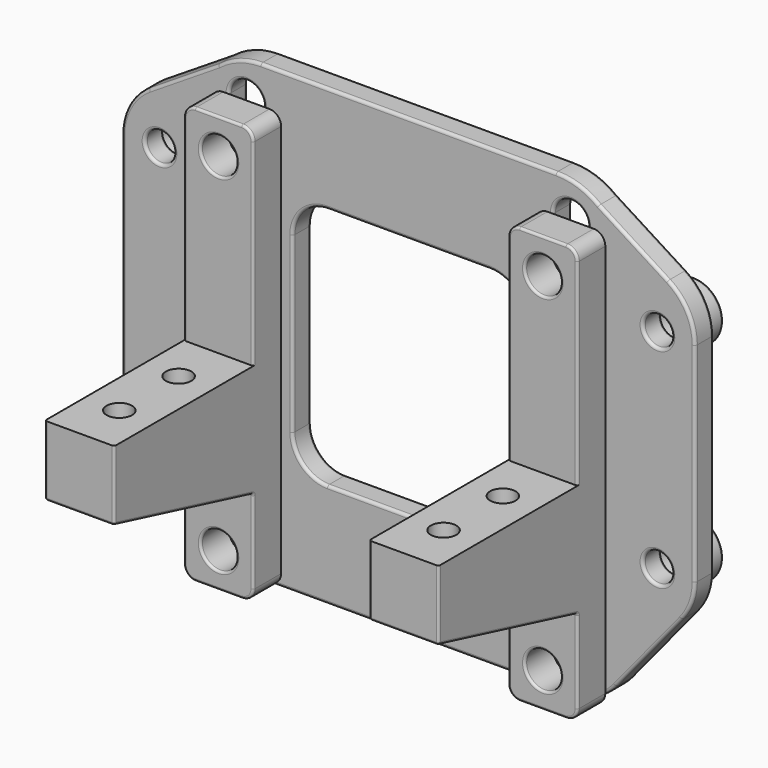
from build123d import *

# Parameters (mm, degrees)
F0_R           = 1.25
F1_DEPTH       = 1
F2_R           = 0.25
F3_R           = 0.25
F4_R           = 2.5046976259
F4_R_2         = 1.5
F5_DEPTH       = 2
F6_R           = 0.25
F7_R           = 1.55
F7_W           = 6
F7_H           = 10
F8_DEPTH       = 3
F9_DEPTH       = 18
F10_T4_DEPTH   = 89.1080799927
F11_R          = 1.1
F12_DEPTH      = 6
F12_DEPTH_BACK = 6
F13_R          = 0.2


# Not quite as in the source:
# - a fillet or chamfer that OpenCascade refuses, or shapes differently, is made with other operations: its cross-section is extruded or revolved along the edge and cut away or added
# - a feature names something its author has since deleted; it is built from what else it names


with BuildPart() as f1:
    # F0 (on Front) → F1 (new body, symmetric)
    with BuildSketch(Plane.XZ):
        with BuildLine():
            Line((12.8879709855, 19.8976094481), (-12.6006863486, 19.8976094481))
            ThreePointArc((-12.6006863486, 19.8976094481), (-14.5633321284, 19.5675319823), (-16.3100361931, 18.6136166291))
            Line((-16.3100361931, 18.6136166291), (-22.2808921813, 14.8335119712))
            ThreePointArc((-22.2808921813, 14.8335119712), (-23.9865787247, 13.0201109666), (-24.6063577035, 10.6089569264))
            Line((-24.6063577035, 10.6089569264), (-24.6063577035, -7.3910430736))
            ThreePointArc((-24.6063577035, -7.3910430736), (-24.3140186875, -9.0756581809), (-23.4711864795, -10.5632817991))
            Line((-23.4711864795, -10.5632817991), (-17.7714078324, -17.5074844391))
            ThreePointArc((-17.7714078324, -17.5074844391), (-16.0441952956, -18.855267485), (-13.9065790564, -19.3352457136))
            Line((-13.9065790564, -19.3352457136), (14.1938643656, -19.3352457136))
            ThreePointArc((14.1938643656, -19.3352457136), (16.3314807451, -18.8552674187), (18.0586933385, -17.5074841993))
            Line((18.0586933385, -17.5074841993), (23.7584712695, -10.5632815531))
            ThreePointArc((23.7584712695, -10.5632815531), (24.6013033328, -9.0756580287), (24.8936422965, -7.3910430674))
            Line((24.8936422965, -7.3910430674), (24.8936422965, 10.6089569326))
            ThreePointArc((24.8936422965, 10.6089569326), (24.2738633208, 13.0201109671), (22.5681767852, 14.8335119706))
            Line((22.5681767852, 14.8335119706), (16.59732083, 18.6136166291))
            ThreePointArc((16.59732083, 18.6136166291), (14.8506167653, 19.5675319823), (12.8879709855, 19.8976094481))
        make_face()
        with BuildLine():
            Line((-15.3563577035, -16.316389355), (-15.3563577035, -13.316389355))
            ThreePointArc((-15.3563577035, -13.316389355), (-13.8563577035, -11.816389355), (-12.3563577035, -13.316389355))
            Line((-12.3563577035, -13.316389355), (-12.3563577035, -16.316389355))
            ThreePointArc((-12.3563577035, -16.316389355), (-13.8563577035, -17.816389355), (-15.3563577035, -16.316389355))
        make_face(mode=Mode.SUBTRACT)
        with Locations((-21.3563577035, -7.316389355)):
            Circle(F0_R, mode=Mode.SUBTRACT)
        with BuildLine():
            Line((12.6436422965, -16.316389355), (12.6436422965, -13.316389355))
            ThreePointArc((12.6436422965, -13.316389355), (14.1436422965, -11.816389355), (15.6436422965, -13.316389355))
            Line((15.6436422965, -13.316389355), (15.6436422965, -16.316389355))
            ThreePointArc((15.6436422965, -16.316389355), (14.1436422965, -17.816389355), (12.6436422965, -16.316389355))
        make_face(mode=Mode.SUBTRACT)
        with BuildLine():
            Line((-9.8563577035, -7.316389355), (-9.8563577035, 7.683610645))
            ThreePointArc((-9.8563577035, 7.683610645), (-8.977678047, 9.8049309885), (-6.8563577035, 10.683610645))
            Line((-6.8563577035, 10.683610645), (7.1436422965, 10.683610645))
            ThreePointArc((7.1436422965, 10.683610645), (9.2649626401, 9.8049309885), (10.1436422965, 7.683610645))
            Line((10.1436422965, 7.683610645), (10.1436422965, -7.316389355))
            ThreePointArc((10.1436422965, -7.316389355), (9.2649626401, -9.4377096986), (7.1436422965, -10.316389355))
            Line((7.1436422965, -10.316389355), (-6.8563577035, -10.316389355))
            ThreePointArc((-6.8563577035, -10.316389355), (-8.977678047, -9.4377096986), (-9.8563577035, -7.316389355))
        make_face(mode=Mode.SUBTRACT)
        with Locations((21.6436422965, -7.316389355)):
            Circle(F0_R, mode=Mode.SUBTRACT)
        with Locations((-21.3563577035, 10.683610645)):
            Circle(F0_R, mode=Mode.SUBTRACT)
        with BuildLine():
            Line((-15.3563577035, 13.683610645), (-15.3563577035, 16.683610645))
            ThreePointArc((-15.3563577035, 16.683610645), (-13.8563577035, 18.183610645), (-12.3563577035, 16.683610645))
            Line((-12.3563577035, 16.683610645), (-12.3563577035, 13.683610645))
            ThreePointArc((-12.3563577035, 13.683610645), (-13.8563577035, 12.183610645), (-15.3563577035, 13.683610645))
        make_face(mode=Mode.SUBTRACT)
        with Locations((21.6436422965, 10.683610645)):
            Circle(F0_R, mode=Mode.SUBTRACT)
        with BuildLine():
            Line((12.6436422965, 13.683610645), (12.6436422965, 16.683610645))
            ThreePointArc((12.6436422965, 16.683610645), (14.1436422965, 18.183610645), (15.6436422965, 16.683610645))
            Line((15.6436422965, 16.683610645), (15.6436422965, 13.683610645))
            ThreePointArc((15.6436422965, 13.683610645), (14.1436422965, 12.183610645), (12.6436422965, 13.683610645))
        make_face(mode=Mode.SUBTRACT)
    extrude(amount=F1_DEPTH, both=True)

    # F2
    f2_edges = [f1.edges().sort_by_distance(p)[0] for p in [
        (24.893642, -1, 1.608957),
        (24.273863, -1, 13.020111),
        (19.582749, -1, 16.723564),
        (14.850617, -1, 19.567532),
        (0.143642, -1, 19.897609),
        (-14.563332, -1, 19.567532),
        (-19.295464, -1, 16.723564),
        (-23.986579, -1, 13.020111),
        (-24.606358, -1, 1.608957),
        (-24.314019, -1, -9.075658),
        (-20.621297, -1, -14.035383),
        (-16.044195, -1, -18.855267),
        (0.143643, -1, -19.335246),
        (16.331481, -1, -18.855267),
        (20.908582, -1, -14.035383),
        (24.601303, -1, -9.075658),
        (-13.856358, -1, -17.816389),
        (-15.356358, -1, -14.816389),
        (-13.856358, -1, -11.816389),
        (-12.356358, -1, -14.816389),
        (-22.606358, -1, -7.316389),
        (15.643642, -1, -14.816389),
        (14.143642, -1, -17.816389),
        (12.643642, -1, -14.816389),
        (14.143642, -1, -11.816389),
        (0.143642, -1, -10.316389),
        (-8.977678, -1, -9.43771),
        (-9.856358, -1, 0.183611),
        (-8.977678, -1, 9.804931),
        (0.143642, -1, 10.683611),
        (9.264963, -1, 9.804931),
        (10.143642, -1, 0.183611),
        (9.264963, -1, -9.43771),
        (20.393642, -1, -7.316389),
        (-22.606358, -1, 10.683611),
        (-12.356358, -1, 15.183611),
        (-13.856358, -1, 12.183611),
        (-15.356358, -1, 15.183611),
        (-13.856358, -1, 18.183611),
        (20.393642, -1, 10.683611),
        (14.143642, -1, 12.183611),
        (12.643642, -1, 15.183611),
        (14.143642, -1, 18.183611),
        (15.643642, -1, 15.183611),
    ]]
    fillet(f2_edges, radius=F2_R)

    # F3
    f3_edges = [f1.edges().sort_by_distance(p)[0] for p in [
        (24.893642, 1, 1.608957),
        (24.273863, 1, 13.020111),
        (19.582749, 1, 16.723564),
        (14.850617, 1, 19.567532),
        (0.143642, 1, 19.897609),
        (-14.563332, 1, 19.567532),
        (-19.295464, 1, 16.723564),
        (-23.986579, 1, 13.020111),
        (-24.606358, 1, 1.608957),
        (-24.314019, 1, -9.075658),
        (-20.621297, 1, -14.035383),
        (-16.044195, 1, -18.855267),
        (0.143643, 1, -19.335246),
        (16.331481, 1, -18.855267),
        (20.908582, 1, -14.035383),
        (24.601303, 1, -9.075658),
        (-13.856358, 1, -17.816389),
        (-15.356358, 1, -14.816389),
        (-13.856358, 1, -11.816389),
        (-12.356358, 1, -14.816389),
        (-22.606358, 1, -7.316389),
        (15.643642, 1, -14.816389),
        (14.143642, 1, -17.816389),
        (12.643642, 1, -14.816389),
        (14.143642, 1, -11.816389),
        (0.143642, 1, -10.316389),
        (-8.977678, 1, -9.43771),
        (-9.856358, 1, 0.183611),
        (-8.977678, 1, 9.804931),
        (0.143642, 1, 10.683611),
        (9.264963, 1, 9.804931),
        (10.143642, 1, 0.183611),
        (9.264963, 1, -9.43771),
        (20.393642, 1, -7.316389),
        (-22.606358, 1, 10.683611),
        (-12.356358, 1, 15.183611),
        (-13.856358, 1, 12.183611),
        (-15.356358, 1, 15.183611),
        (-13.856358, 1, 18.183611),
        (20.393642, 1, 10.683611),
        (14.143642, 1, 12.183611),
        (12.643642, 1, 15.183611),
        (14.143642, 1, 18.183611),
        (15.643642, 1, 15.183611),
    ]]
    fillet(f3_edges, radius=F3_R)

    # F4 (on face) → F5 (join)
    with BuildSketch(Plane(origin=(0, 1, 0), x_dir=(-1, 0, 0), z_dir=(0, 1, 0))):
        with Locations((-21.6436422965, 10.683610645)):
            Circle(F4_R)
        with Locations((-21.6436422965, 10.683610645)):
            Circle(F4_R_2, mode=Mode.SUBTRACT)
        with Locations((-21.6436422965, -7.316389355)):
            Circle(F4_R)
        with Locations((-21.6436422965, -7.316389355)):
            Circle(F4_R_2, mode=Mode.SUBTRACT)
        with Locations((21.3563577035, -7.316389355)):
            Circle(F4_R)
        with Locations((21.3563577035, -7.316389355)):
            Circle(F4_R_2, mode=Mode.SUBTRACT)
        with Locations((21.3563577035, 10.683610645)):
            Circle(F4_R)
        with Locations((21.3563577035, 10.683610645)):
            Circle(F4_R_2, mode=Mode.SUBTRACT)
    extrude(amount=F5_DEPTH)

    # F6
    f6_edges = [f1.edges().sort_by_distance(p)[0] for p in [
        (-18.85166, 3, 10.683611),
        (-19.856358, 3, 10.683611),
        (24.14834, 3, 10.683611),
        (23.143642, 3, 10.683611),
        (24.14834, 3, -7.316389),
        (23.143642, 3, -7.316389),
        (-19.856358, 3, -7.316389),
        (-18.85166, 3, -7.316389),
    ]]
    fillet(f6_edges, radius=F6_R)


with BuildPart() as f8:
    # F7 (on face) → F8 (new body)
    with BuildSketch(Plane.XZ.offset(1)):
        with BuildLine():
            Line((-11.8563577035, 16.683610645), (-15.8563577035, 16.683610645))
            ThreePointArc((-15.8563577035, 16.683610645), (-16.5634644846, 16.3907174262), (-16.8563577035, 15.683610645))
            Line((-16.8563577035, 15.683610645), (-16.8563577035, -1.316389355))
            Line((-16.8563577035, -1.316389355), (-10.8563577035, -1.316389355))
            Line((-10.8563577035, -1.316389355), (-10.8563577035, 15.683610645))
            ThreePointArc((-10.8563577035, 15.683610645), (-11.1492509223, 16.3907174262), (-11.8563577035, 16.683610645))
        make_face()
        with Locations((-13.8563577035, 13.683610645)):
            Circle(F7_R, mode=Mode.SUBTRACT)
        with Locations((-13.8563577035, -6.316389355)):
            Rectangle(F7_W, F7_H)
        with BuildLine():
            Line((-10.8563577035, -11.316389355), (-16.8563577035, -11.316389355))
            Line((-16.8563577035, -11.316389355), (-16.8563577035, -18.316389355))
            ThreePointArc((-16.8563577035, -18.316389355), (-16.5634644846, -19.0234961362), (-15.8563577035, -19.316389355))
            Line((-15.8563577035, -19.316389355), (-11.8563577035, -19.316389355))
            ThreePointArc((-11.8563577035, -19.316389355), (-11.1492509223, -19.0234961362), (-10.8563577035, -18.316389355))
            Line((-10.8563577035, -18.316389355), (-10.8563577035, -11.316389355))
        make_face()
        with Locations((-13.8563577035, -16.316389355)):
            Circle(F7_R, mode=Mode.SUBTRACT)
    extrude(amount=F8_DEPTH)

    # F7 (on face) → F9 (join)
    with BuildSketch(Plane.XZ.offset(1)):
        with Locations((-13.8563577035, -6.316389355)):
            Rectangle(F7_W, F7_H)
    extrude(amount=F9_DEPTH)

    # F10: chamfer of 4 x 16 on 1 edges, made by hand


with BuildPart() as f10_tool2:
    # F10_s3 → F10_t4 (new body)
    with BuildSketch(Plane.YZ.offset(-58.4103976998)):
        Polygon((-3, -11.316389355), (-19, -7.316389355), (-19, -11.316389355), align=None)
    extrude(amount=F10_T4_DEPTH)

    split(bisect_by=Plane.XZ.offset(4), keep=Keep.TOP)


with BuildPart() as f8_1:
    add(f8.part)

    # F10_t1: cut F10_tool2
    add(f10_tool2.part, mode=Mode.SUBTRACT)

    # F11 (on face) → F12 (cut, two sides)
    with BuildSketch(Plane.XY.offset(-1.316389355)) as f12_sk:
        with Locations((-13.8654727489, -8.3)):
            Circle(F11_R)
        with Locations((-13.8654727489, -14.7)):
            Circle(F11_R)
    extrude(amount=-F12_DEPTH, mode=Mode.SUBTRACT)
    extrude(f12_sk.sketch, amount=F12_DEPTH_BACK, mode=Mode.SUBTRACT)

    # F13
    f13_edges = [f8_1.edges().sort_by_distance(p)[0] for p in [
        (-16.856358, -11.5, -9.191389),
        (-13.856358, -19, -7.316389),
        (-10.856358, -11.5, -9.191389),
        (-13.856358, -4, -11.066389),
        (-16.856358, -19, -4.316389),
        (-10.856358, -19, -4.316389),
        (-16.856358, -4, 7.183611),
        (-15.406358, -4, 13.683611),
        (-15.406358, -4, -16.316389),
        (-11.149251, -4, 16.390717),
        (-10.856358, -4, -14.691389),
        (-10.856358, -4, 7.183611),
        (-13.856358, -4, 16.683611),
        (-16.563464, -4, 16.390717),
        (-11.149251, -4, -19.023496),
        (-16.856358, -4, -14.691389),
        (-16.563464, -4, -19.023496),
        (-13.856358, -4, -19.316389),
    ]]
    fillet(f13_edges, radius=F13_R)


with BuildPart() as f14_1:
    # F14: copy of F8
    add(f8_1.part.moved(Location((28, 0, 0))))


solid = Compound([f1.part, f8_1.part, f14_1.part])
